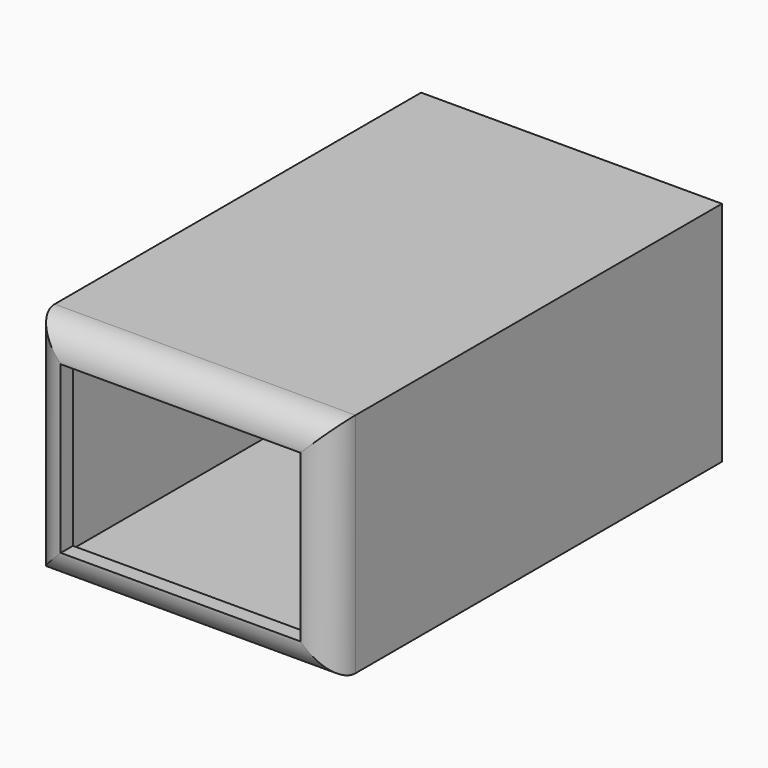
from build123d import *

# Parameters (mm, degrees)
F0_W     = 50.0364415348
F0_H     = 37.788476795
F1_DEPTH = 81.28
F2_R     = 5.08
F3_T     = -2.54


# Not quite as in the source:
# - a shell that OpenCascade refuses in one call is made with other operations: the cavity is built on its own and cut out


with BuildPart() as f1:
    # F0 (on Front) → F1 (new body)
    with BuildSketch(Plane.XZ):
        with Locations((25.0182207674, -18.8942383975)):
            Rectangle(F0_W, F0_H)
    extrude(amount=F1_DEPTH)

    # F2
    f2_edges = [f1.edges().sort_by_distance(p)[0] for p in [
        (25.018221, -81.28, 0),
        (0, -81.28, -18.894238),
        (25.018221, -81.28, -37.788477),
        (50.036442, -81.28, -18.894238),
    ]]
    fillet(f2_edges, radius=F2_R)

    # F3: a shell. OpenCascade refuses it in one call, so the cavity is built on its own and cut out:
    # the body offset inwards by the wall thickness, plus a prism from it out through each open face.
    f3_core = offset(f1.part, amount=F3_T, mode=Mode.PRIVATE)
    f3_exits = [f3_core.faces().sort_by_distance(p)[0] for p in [
        (25.018221, -78.74, -18.894238),
    ]]
    add(f3_core, mode=Mode.SUBTRACT)
    extrude(f3_exits, amount=-F3_T, mode=Mode.SUBTRACT)


solid = f1.part
